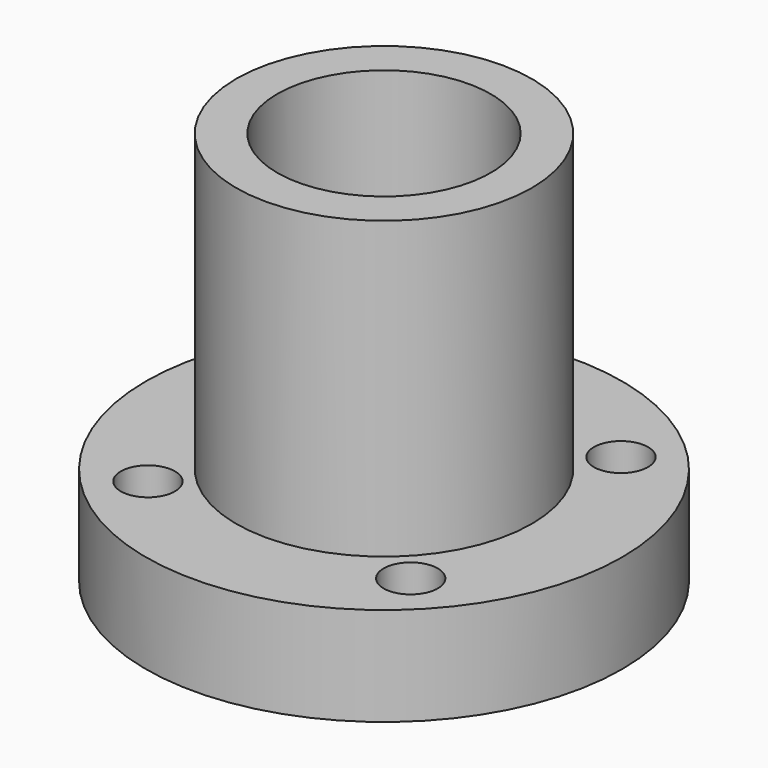
from build123d import *

# Parameters (mm, degrees)
F0_R     = 14.5
F0_R_2   = 9
F1_DEPTH = 6
F2_DEPTH = 18
F4_D     = 13
F6_D     = 3.3


with BuildPart() as f1:
    # F0 (on Top) → F1 (new body)
    with BuildSketch(Plane.XY):
        Circle(F0_R)
        Circle(F0_R_2, mode=Mode.SUBTRACT)
        Circle(F0_R_2)
    extrude(amount=-F1_DEPTH)

    # F0 (on Top) → F2 (join)
    with BuildSketch(Plane.XY):
        Circle(F0_R_2)
    extrude(amount=F2_DEPTH)

    # F4 (through all)
    with Locations(Plane.XY.offset(18)):
        with Locations((0, 0)):
            Hole(F4_D / 2)

    # F6 (through all)
    with Locations(Plane(origin=(0, 0, -6), x_dir=(1, 0, 0), z_dir=(0, 0, -1))):
        with Locations((8.0136820347, 7.9841035315), (8.0136820347, -8.0158964685), (-7.9863179653, -8.0158964685), (-7.9863179653, 7.9841035315)):
            Hole(F6_D / 2)


solid = f1.part
